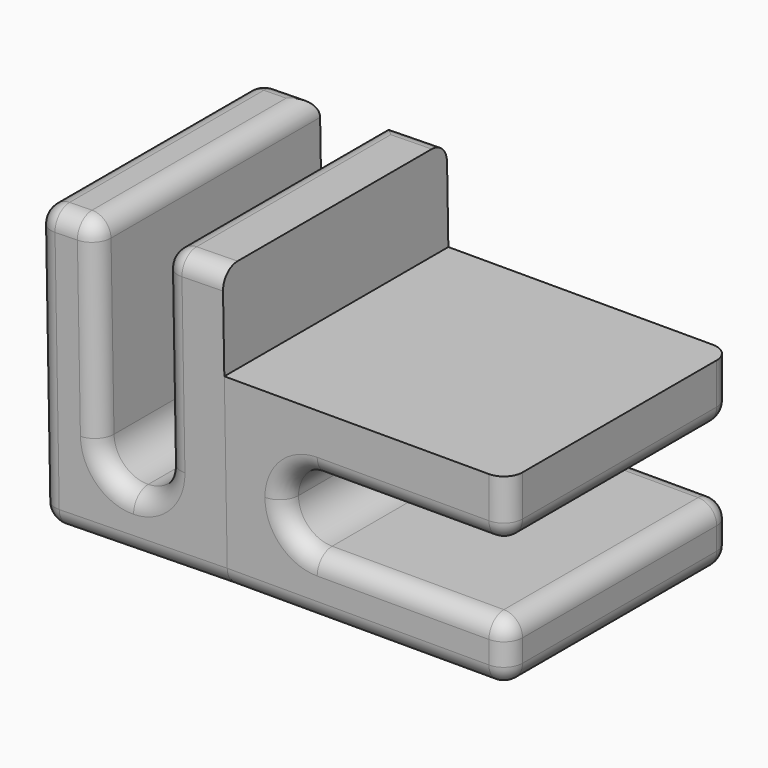
from build123d import *

# Parameters (mm, degrees)
F0_W     = 15
F0_H     = 15
F1_DEPTH = 10
F2_W     = 15
F2_H     = 3.6
F3_DEPTH = 12
F4_R     = 1.79999
F5_COUNT = 2
F5_ANGLE = 91
F7_DEPTH = 15
F8_R     = 1
F8_2_R   = 1


# Not quite as in the source:
# - a fillet or chamfer is up to 0.001 mm smaller than in the source, because OpenCascade refuses the exact size


with BuildPart() as f1:
    # F0 (on Top) → F1 (new body)
    with BuildSketch(Plane.XY):
        with Locations((7.5, 7.5)):
            Rectangle(F0_W, F0_H)
    extrude(amount=F1_DEPTH)

    # F2 (on face) → F3 (cut)
    with BuildSketch(Plane.YZ.offset(15)):
        with Locations((7.5, 5)):
            Rectangle(F2_W, F2_H)
    extrude(amount=-F3_DEPTH, mode=Mode.SUBTRACT)

    # F4 (radius 1.8 in the source; OpenCascade refuses exactly that, so slightly less here)
    f4_edges = [f1.edges().sort_by_distance(p)[0] for p in [
        (3, 7.5, 3.2),
        (3, 7.5, 6.8),
    ]]
    fillet(f4_edges, radius=F4_R)


with BuildPart() as f5_1:
    # F5: instance of F1
    add(f1.part.rotate(Axis((0, 7.5, 0), (0, -1, 0)), 1 * F5_ANGLE / (F5_COUNT - 1)))

    # F8#2
    f8_2_edges = [f5_1.edges().sort_by_distance(p)[0] for p in [
        (-10.12937, 0, 7.324334),
        (-6.971743, 0, 9.779811),
        (-8.660507, 0, 14.851115),
        (-7.06075, 7.5, 14.879039),
        (-8.660507, 15, 14.851115),
        (-10.260263, 7.5, 14.823191),
        (-9.998477, 7.5, -0.174524),
        (-10.12937, 15, 7.324334),
        (-3.461299, 7.5, 14.941868),
        (-4.999238, 0, -0.087262),
        (-4.999238, 15, -0.087262),
        (-1.861542, 0, 14.969792),
        (-1.861542, 15, 14.969792),
        (-6.333398, 0, 3.417192),
        (-5.051596, 0, 2.912281),
        (-3.788195, 0, 3.461619),
        (-3.372291, 0, 9.842639),
    ]]
    fillet(f8_2_edges, radius=F8_2_R)


with BuildPart() as f1_1:
    add(f1.part)

    # F6 (on face) → F7 (join, through all)
    with BuildSketch(Plane.XZ):
        Polygon((0, 0), (0, 10), (-0.1745506493, 10), align=None)
    extrude(amount=-F7_DEPTH)

    # F8
    f8_edges = [f1_1.edges().sort_by_distance(p)[0] for p in [
        (9.899995, 0, 6.8),
        (15, 7.5, 6.8),
        (15, 15, 1.6),
        (15, 0, 1.6),
        (15, 7.5, 3.2),
        (9.899995, 15, 3.2),
        (15, 7.5, 0),
        (7.5, 0, 0),
        (7.5, 15, 0),
        (15, 0, 8.4),
        (15, 15, 8.4),
        (9.899995, 15, 6.8),
        (3.527205, 15, 3.727205),
        (3, 15, 5),
        (3.527205, 15, 6.272795),
        (3.527205, 0, 6.272795),
        (9.899995, 0, 3.2),
        (3, 0, 5),
        (3.527205, 0, 3.727205),
    ]]
    fillet(f8_edges, radius=F8_R)


solid = Compound([f5_1.part, f1_1.part])
